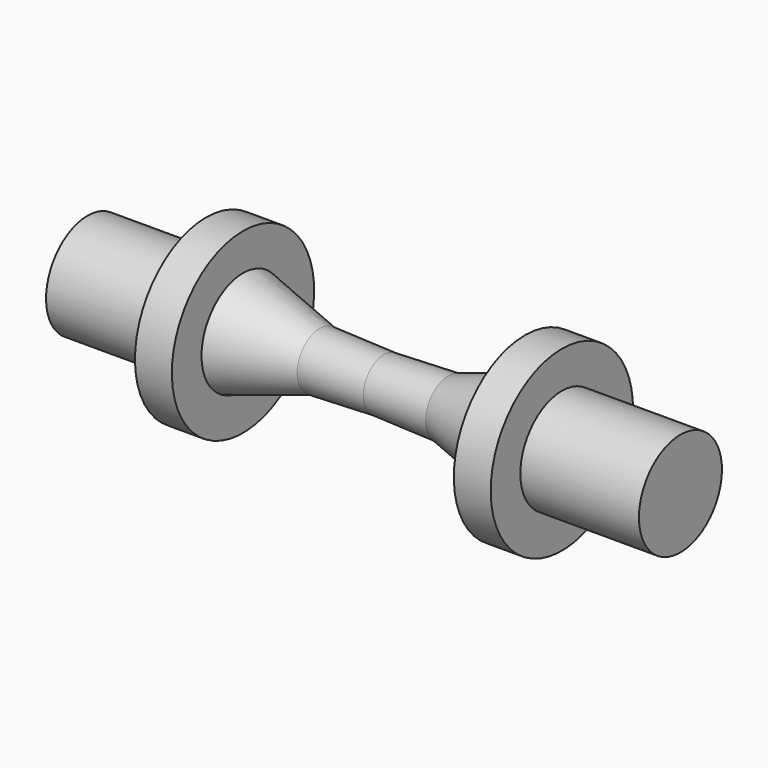
from build123d import *


with BuildPart() as f1:
    # F0 (on Front) → F1 (revolve)
    with BuildSketch(Plane.XZ):
        with BuildLine():
            Line((47.5609842221, 30), (47.5609842221, 17.5))
            add(Edge.make_bspline(
                [(21.6804631054, 9.5182526857), (30.3073034776, 12.1788351238), (38.9341438499, 14.8394175619), (47.5609842221, 17.5)],
                knots=[0, 0, 0, 0, 27.0833835305, 27.0833835305, 27.0833835305, 27.0833835305], degree=3))
            add(Edge.make_bspline(
                [(21.6804631054, 9.5182526857), (14.4536420703, 9.2621684571), (7.2268210351, 9.0060842286), (0, 8.75)],
                knots=[0, 0, 0, 0, 21.6940704492, 21.6940704492, 21.6940704492, 21.6940704492], degree=3))
            Line((0, 8.75), (0, 0))
            Line((0, 0), (100, 0))
            Line((100, 0), (100, 17.5))
            Line((100, 17.5), (60, 17.5))
            Line((60, 17.5), (60, 30))
            Line((60, 30), (47.5609842221, 30))
        make_face()
    revolve(axis=Axis((50, 0, 0), (1, 0, 0)))

    # F2: F1 across face


with BuildPart() as f1_1:
    add(f1.part)
    add(f1.part.mirror(Plane(origin=(0, 0, 0), x_dir=(0, -1, 0), z_dir=(-1, 0, 0))))


solid = f1_1.part
